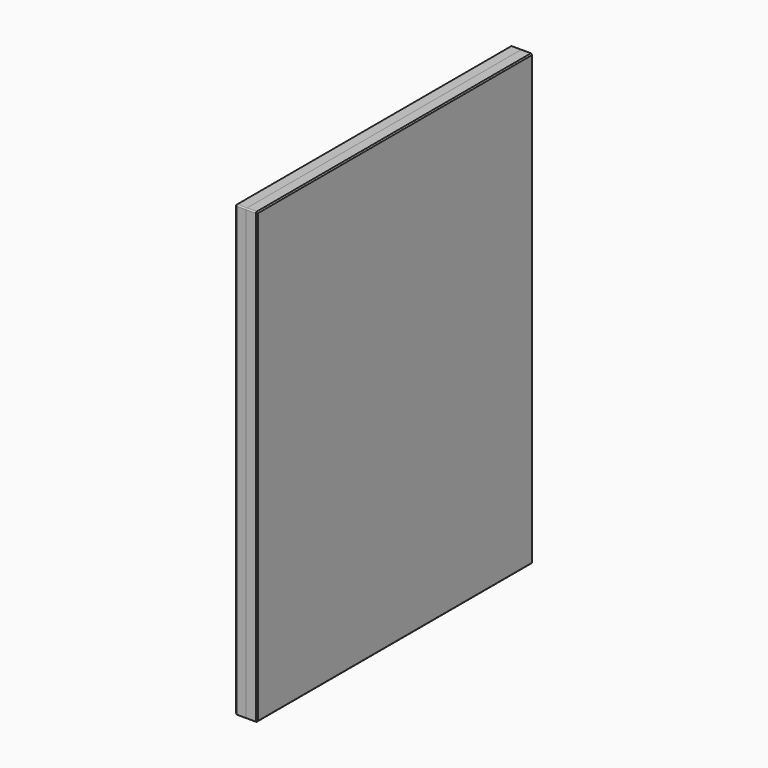
from build123d import *

# Parameters (mm, degrees)
F1_DEPTH = 19
F2_SIZE2 = 1.99999
F2_SIZE  = 1.99999


# Not quite as in the source:
# - a fillet or chamfer is up to 0.001 mm smaller than in the source, because OpenCascade refuses the exact size


with BuildPart() as f1:
    # F0 (on Right) → F1 (new body)
    with BuildSketch(Plane.YZ):
        with BuildLine():
            Line((298, 391), (-298, 391))
            ThreePointArc((-298, 391), (-299.4142135624, 390.4142135624), (-300, 389))
            Line((-300, 389), (-300, -389))
            ThreePointArc((-300, -389), (-299.4142135624, -390.4142135624), (-298, -391))
            Line((-298, -391), (298, -391))
            ThreePointArc((298, -391), (299.4142135624, -390.4142135624), (300, -389))
            Line((300, -389), (300, 389))
            ThreePointArc((300, 389), (299.4142135624, 390.4142135624), (298, 391))
        make_face()
    extrude(amount=F1_DEPTH)

    # F2 (size 2 and 2 in the source; OpenCascade refuses exactly that, so slightly less here)
    f2_edges = [f1.edges().sort_by_distance(p)[0] for p in [
        (0, 0, 391),
        (0, -300, 0),
        (0, 0, -391),
        (0, 300, 0),
    ]]
    chamfer(f2_edges, length=F2_SIZE, length2=F2_SIZE2)


with BuildPart() as f3_1:
    # F3: instance of F1
    add(f1.part.mirror(Plane.YZ.offset(19)))


solid = Compound([f1.part, f3_1.part])
